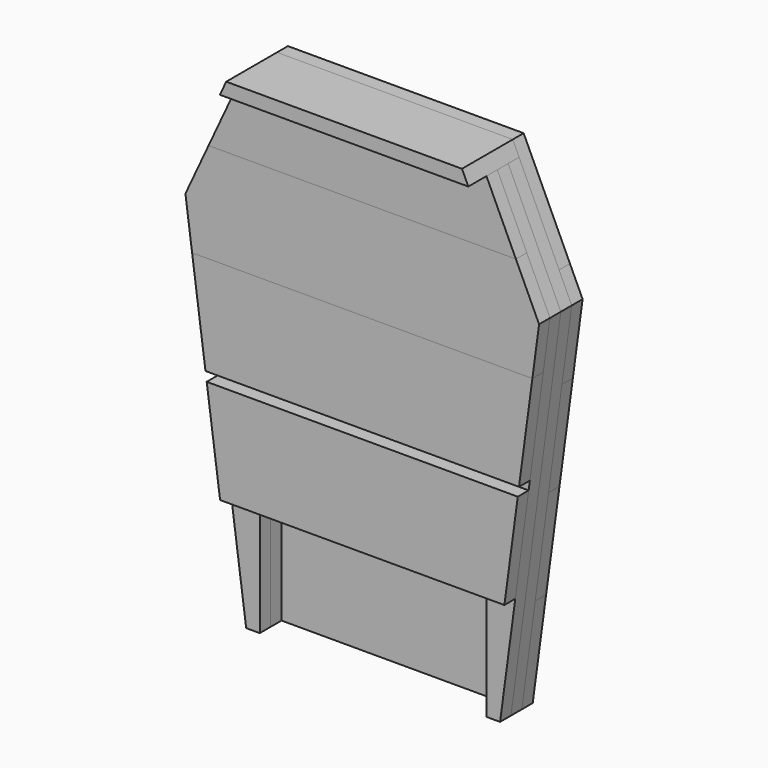
from build123d import *

# Parameters (mm, degrees)
F2_DEPTH  = 19.05
F3_DEPTH  = 19.05
F5_DEPTH  = 19.05
F7_DEPTH  = 19.05
F8_DEPTH  = 88.9
F10_DEPTH = 19.05
F11_DEPTH = 19.05


# Not quite as in the source:
# - a feature names something its author has since deleted; it is built from what else it names


with BuildPart() as f2:
    # F1 (on Front) → F2 (new body)
    with BuildSketch(Plane.XZ):
        Polygon((-215.2804878049, -419.1), (-196.5402439024, -558.8), (196.5402439024, -558.8), (215.2804878049, -419.1), align=None)
    extrude(amount=F2_DEPTH)


with BuildPart() as f2b:
    # F1 (on Front) → F2, piece 2 (new body)
    with BuildSketch(Plane.XZ):
        Polygon((-247.65, -177.8), (-234.0207317073, -279.4), (234.0207317073, -279.4), (247.65, -177.8), (229.9607142857, -139.7), (-229.9607142857, -139.7), align=None)
    extrude(amount=F2_DEPTH)


with BuildPart() as f3:
    # F1 (on Front) → F3 (new body)
    with BuildSketch(Plane.XZ):
        Polygon((-196.5402439024, -558.8), (-177.8, -698.5), (177.8, -698.5), (196.5402439024, -558.8), align=None)
    extrude(amount=F3_DEPTH)


with BuildPart() as f3b:
    # F1 (on Front) → F3, piece 2 (new body)
    with BuildSketch(Plane.XZ):
        Polygon((-234.0207317073, -279.4), (-215.2804878049, -419.1), (215.2804878049, -419.1), (234.0207317073, -279.4), align=None)
    extrude(amount=F3_DEPTH)


with BuildPart() as f3c:
    # F1 (on Front) → F3, piece 3 (new body)
    with BuildSketch(Plane.XZ):
        Polygon((-165.1, 0), (-229.9607142857, -139.7), (229.9607142857, -139.7), (165.1, 0), align=None)
    extrude(amount=F3_DEPTH)


with BuildPart() as f5:
    # F4 (on face) → F5 (new body)
    with BuildSketch(Plane.XZ.offset(19.05)):
        Polygon((-173.9446428571, -19.05), (-229.9607142857, -139.7), (-158.75, -139.7), (-158.75, -19.05), align=None)
        Polygon((-247.65, -177.8), (-177.8, -698.5), (-158.75, -698.5), (-158.75, -139.7), (-229.9607142857, -139.7), align=None)
    extrude(amount=F5_DEPTH)


with BuildPart() as f5b:
    # F4 (on face) → F5, piece 2 (new body)
    with BuildSketch(Plane.XZ.offset(19.05)):
        Polygon((158.75, -19.05), (158.75, -139.7), (229.9607142857, -139.7), (173.9446428571, -19.05), align=None)
        Polygon((229.9607142857, -139.7), (158.75, -139.7), (158.75, -698.5), (177.8, -698.5), (247.65, -177.8), align=None)
    extrude(amount=F5_DEPTH)


with BuildPart() as f7:
    # F6 (on face) → F7 (new body)
    with BuildSketch(Plane.XZ.offset(38.1)):
        Polygon((-247.65, -177.8), (-177.8, -698.5), (-158.75, -698.5), (-158.75, -19.05), (-173.9446428571, -19.05), align=None)
    extrude(amount=F7_DEPTH)


with BuildPart() as f7b:
    # F6 (on face) → F7, piece 2 (new body)
    with BuildSketch(Plane.XZ.offset(38.1)):
        Polygon((173.9446428571, -19.05), (158.75, -19.05), (158.75, -698.5), (177.8, -698.5), (247.65, -177.8), align=None)
    extrude(amount=F7_DEPTH)


with BuildPart() as f8:
    # F4 (on face) → F8 (new body)
    with BuildSketch(Plane.XZ.offset(19.05)):
        Polygon((-165.1, 0), (-173.9446428571, -19.05), (-158.75, -19.05), (158.75, -19.05), (173.9446428571, -19.05), (165.1, 0), align=None)
    extrude(amount=F8_DEPTH)


with BuildPart() as f10:
    # F9 (on face) → F10 (new body)
    with BuildSketch(Plane.XZ.offset(57.15)):
        Polygon((158.75, -107.95), (-215.2196428571, -107.95), (-247.65, -177.8), (-238.2798780488, -247.65), (158.75, -247.65), align=None)
        Polygon((215.2196428571, -107.95), (158.75, -107.95), (158.75, -247.65), (238.2798780488, -247.65), (247.65, -177.8), align=None)
    extrude(amount=F10_DEPTH)


with BuildPart() as f10b:
    # F9 (on face) → F10, piece 2 (new body)
    with BuildSketch(Plane.XZ.offset(57.15)):
        Polygon((158.75, -539.75), (158.75, -400.05), (-217.8359756098, -400.05), (-199.0957317073, -539.75), align=None)
        Polygon((217.8359756098, -400.05), (158.75, -400.05), (158.75, -539.75), (199.0957317073, -539.75), align=None)
    extrude(amount=F10_DEPTH)


with BuildPart() as f11:
    # F9 (on face) → F11 (new body)
    with BuildSketch(Plane.XZ.offset(57.15)):
        Polygon((158.75, -387.35), (158.75, -247.65), (-238.2798780488, -247.65), (-219.5396341463, -387.35), align=None)
        Polygon((238.2798780488, -247.65), (158.75, -247.65), (158.75, -387.35), (219.5396341463, -387.35), align=None)
    extrude(amount=F11_DEPTH)


with BuildPart() as f11b:
    # F9 (on face) → F11, piece 2 (new body)
    with BuildSketch(Plane.XZ.offset(57.15)):
        Polygon((158.75, -19.05), (-173.9446428571, -19.05), (-215.2196428571, -107.95), (158.75, -107.95), align=None)
        Polygon((173.9446428571, -19.05), (158.75, -19.05), (158.75, -107.95), (215.2196428571, -107.95), align=None)
    extrude(amount=F11_DEPTH)


solid = Compound([f2.part, f2b.part, f3.part, f3b.part, f3c.part, f5.part, f5b.part, f7.part, f7b.part, f8.part, f10.part, f10b.part, f11.part, f11b.part])
